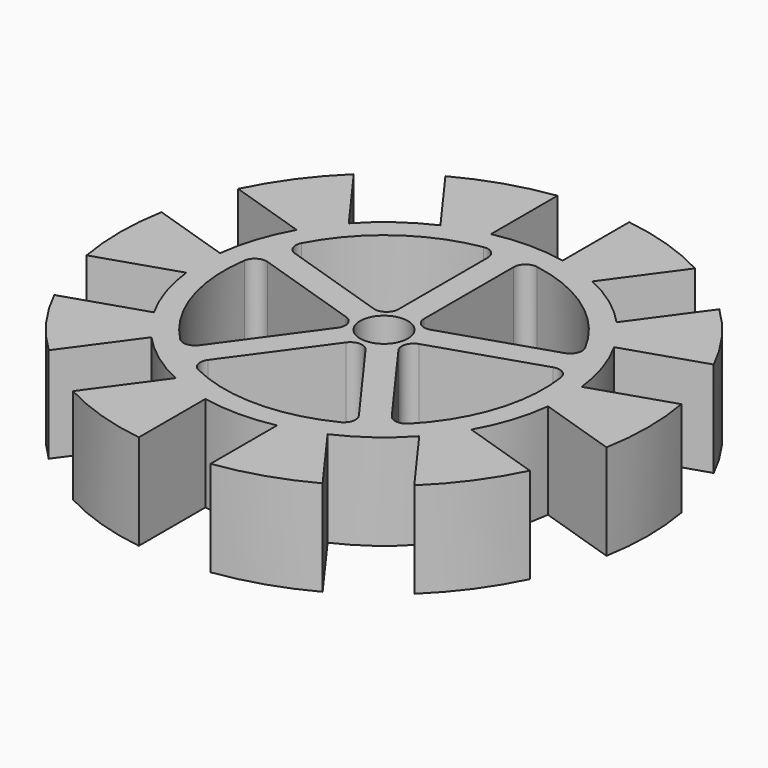
from build123d import *

# Parameters (mm, degrees)
F0_R            = 140.462
F1_DEPTH        = 25.4
F3_DEPTH        = 50.801
F3_COPIES_COUNT = 10
F6_DEPTH        = 50.801
F6_COPIES_COUNT = 5
F7_R            = 12.7
F8_DEPTH        = 50.801


# Not quite as in the source:
# - a pattern or mirror of a feature is missing from the dataset's text; its kind, count and spacing are read off the source's solid


with BuildPart() as f1:
    # F0 (on Top) → F1 (new body, symmetric)
    with BuildSketch(Plane.XY):
        Circle(F0_R)
    extrude(amount=F1_DEPTH, both=True)

    # F2 (on face) → F3 (cut, through all)
    with BuildSketch(Plane.XY.offset(25.4)):
        with BuildLine():
            ThreePointArc((-19.05, 94.9452416198), (0, 96.8375), (19.05, 94.9452416198))
            Line((19.05, 94.9452416198), (19.05, 139.1641870023))
            ThreePointArc((19.05, 139.1641870023), (0, 140.462), (-19.05, 139.1641870023))
            Line((-19.05, 139.1641870023), (-19.05, 94.9452416198))
        make_face()
    f3 = extrude(amount=-F3_DEPTH, mode=Mode.SUBTRACT)

    # F3_copies: F3 ×10 about axis
    f3_copies_axis = Axis((0, 0, 0), (0, 0, 1))
    for i in range(1, F3_COPIES_COUNT):
        add(f3.rotate(f3_copies_axis, i * 360 / F3_COPIES_COUNT), mode=Mode.SUBTRACT)

    # F5 (on face) → F6 (cut, through all)
    with BuildSketch(Plane.XY.offset(25.4)):
        with BuildLine():
            ThreePointArc((71.7178399755, 30.4867595727), (75.6356515828, 34.1286194106), (75.3810322275, 39.4716110682))
            ThreePointArc((75.3810322275, 39.4716110682), (50.0146471176, 68.8392560514), (14.2457129032, 83.8890205204))
            ThreePointArc((14.2457129032, 83.8890205204), (9.0855441629, 82.4801026945), (6.8326, 77.6286458547))
            Line((6.8326, 77.6286458547), (6.8326, 18.1442923048))
            ThreePointArc((6.8326, 18.1442923048), (9.4501636479, 13.0070343905), (15.1448579143, 12.1050834263))
            Line((15.1448579143, 12.1050834263), (71.7178399755, 30.4867595727))
        make_face()
    f6 = extrude(amount=-F6_DEPTH, mode=Mode.SUBTRACT)

    # F6_copies: F6 ×5 about axis
    f6_copies_axis = Axis((0, 0, 0), (0, 0, 1))
    for i in range(1, F6_COPIES_COUNT):
        add(f6.rotate(f6_copies_axis, i * 360 / F6_COPIES_COUNT), mode=Mode.SUBTRACT)

    # F7 (on face) → F8 (cut, through all)
    with BuildSketch(Plane.XY.offset(25.4)):
        Circle(F7_R)
    extrude(amount=-F8_DEPTH, mode=Mode.SUBTRACT)


solid = f1.part
